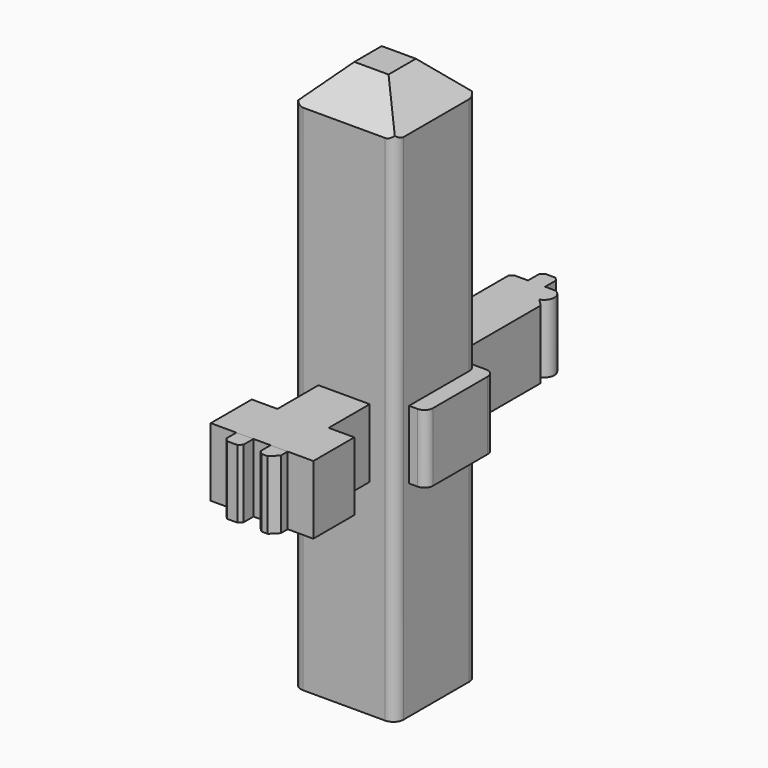
from build123d import *

# Parameters (mm, degrees)
F1_DEPTH      = 25.4
F2_SIZE       = 1.27
F4_DEPTH      = 25.4
F5_SIZE       = 1.27
F6_R          = 3.175
F7_W          = 38.1
F7_H          = 38.1
F8_DEPTH      = 101.6
F9_R          = 3.81
F10_T1_DEPTH  = 95.8007478943
F10_T3_DEPTH  = 95.8007478943
F10_T8_ANGLE  = 90
F10_T13_ANGLE = 90
F10_T18_ANGLE = 90
F10_T23_ANGLE = 90
F10_T28_ANGLE = 90
F10_T33_ANGLE = 90
F10_T38_ANGLE = 90
F10_T43_ANGLE = 90
F12_DEPTH     = 25.4


# Not quite as in the source:
# - a fillet or chamfer that OpenCascade refuses, or shapes differently, is made with other operations: its cross-section is extruded or revolved along the edge and cut away or added


with BuildPart() as f1:
    # F0 (on Top) → F1 (new body)
    with BuildSketch(Plane.XY):
        with BuildLine():
            Line((-3.175, -63.0320869496), (-3.175, -55.4120869496))
            Line((-3.175, -55.4120869496), (3.175, -55.4120869496))
            Line((3.175, -55.4120869496), (3.175, -63.0320869496))
            Line((3.175, -63.0320869496), (6.8309231637, -63.0320869496))
            Line((6.8309231637, -63.0320869496), (9.525, -60.3380101133))
            Line((9.525, -60.3380101133), (9.525, -6.3369898867))
            Line((9.525, -6.3369898867), (6.8309231637, -3.6429130504))
            ThreePointArc((6.8309231637, -3.6429130504), (9.525, 0), (6.8309231637, 3.6429130504))
            Line((6.8309231637, 3.6429130504), (9.525, 6.3369898867))
            Line((9.525, 6.3369898867), (9.525, 60.3380101133))
            Line((9.525, 60.3380101133), (6.8309231637, 63.0320869496))
            ThreePointArc((6.8309231637, 63.0320869496), (9.525, 66.675), (6.8309231637, 70.3179130504))
            Line((6.8309231637, 70.3179130504), (3.175, 70.3179130504))
            Line((3.175, 70.3179130504), (3.175, 76.6679130504))
            Line((3.175, 76.6679130504), (-3.175, 76.6679130504))
            Line((-3.175, 76.6679130504), (-3.175, 70.3179130504))
            Line((-3.175, 70.3179130504), (-9.525, 70.3179130504))
            Line((-9.525, 70.3179130504), (-9.525, -63.0320869496))
            Line((-9.525, -63.0320869496), (-3.175, -63.0320869496))
        make_face()
    extrude(amount=-F1_DEPTH)

    # F2
    f2_edges = [f1.edges().sort_by_distance(p)[0] for p in [
        (-3.175, 76.667913, -12.7),
        (-9.525, 70.317913, -12.7),
        (3.175, 76.667913, -12.7),
        (-9.525, -63.032087, -12.7),
        (-3.175, -63.032087, -12.7),
        (3.175, -63.032087, -12.7),
    ]]
    chamfer(f2_edges, length=F2_SIZE)


with BuildPart() as f4:
    # F3 (on Top) → F4 (new body)
    with BuildSketch(Plane.XY):
        Polygon((0, 19.05), (0, 0), (-12.7, 0), (-12.7, -12.7), (25.4, -12.7), (25.4, 19.05), (12.7, 19.05), (12.7, 25.4), (6.35, 25.4), (6.35, 19.05), align=None)
    extrude(amount=-F4_DEPTH)

    # F5
    f5_edges = [f4.edges().sort_by_distance(p)[0] for p in [
        (12.7, 25.4, -12.7),
        (6.35, 25.4, -12.7),
        (0, 19.05, -12.7),
        (-12.7, 0, -12.7),
    ]]
    chamfer(f5_edges, length=F5_SIZE)

    # F6
    f6_edges = [f4.edges().sort_by_distance(p)[0] for p in [
        (25.4, 19.05, -12.7),
        (25.4, -12.7, -12.7),
    ]]
    fillet(f6_edges, radius=F6_R)


with BuildPart() as f8:
    # F7 (on Top) → F8 (new body, symmetric)
    with BuildSketch(Plane.XY):
        Rectangle(F7_W, F7_H)
    extrude(amount=F8_DEPTH, both=True)

    # F9
    f9_edges = [f8.edges().sort_by_distance(p)[0] for p in [
        (-19.05, -19.05, 0),
        (19.05, -19.05, 0),
        (19.05, 19.05, 0),
        (-19.05, 19.05, 0),
    ]]
    fillet(f9_edges, radius=F9_R)

    # F10: chamfer of 12.7 on 4 edges, made by hand

    # F10_s2 → F10_t1 (cut)
    with BuildSketch(Plane.YZ.offset(-47.9003739472)):
        Polygon((6.35, 101.6), (19.05, 88.9), (19.05, 101.6), align=None)
        Polygon((-19.05, 88.9), (-6.35, 101.6), (-19.05, 101.6), align=None)
    extrude(amount=F10_T1_DEPTH, mode=Mode.SUBTRACT)

    # F10_s4 → F10_t3 (cut)
    with BuildSketch(Plane.XZ.offset(-47.9003739472)):
        Polygon((-6.35, 101.6), (-19.05, 88.9), (-19.05, 101.6), align=None)
        Polygon((6.35, 101.6), (19.05, 88.9), (19.05, 101.6), align=None)
    extrude(amount=F10_T3_DEPTH, mode=Mode.SUBTRACT)


with BuildPart() as f10_tool6:
    # F10_s7 → F10_t8 (revolve)
    with BuildSketch(Plane.YZ.offset(15.24)):
        Polygon((-19.05, 88.9), (-15.24, 92.71), (-15.24, 101.6), (-19.05, 101.6), align=None)
    revolve(axis=Axis((15.24, -15.24, 101.6), (0, 0, 1)), revolution_arc=F10_T8_ANGLE)

    split(bisect_by=Plane(origin=(0, -53.975, 53.975), x_dir=(1, 0, 0), z_dir=(0, -0.7071067812, 0.7071067812)), keep=Keep.TOP)


with BuildPart() as f8_1:
    add(f8.part)

    # F10_t5: cut F10_tool6
    add(f10_tool6.part, mode=Mode.SUBTRACT)


with BuildPart() as f10_tool11:
    # F10_s12 → F10_t13 (revolve)
    with BuildSketch(Plane.YZ.offset(15.24)):
        Polygon((-19.05, 88.9), (-15.24, 92.71), (-15.24, 101.6), (-19.05, 101.6), align=None)
    revolve(axis=Axis((15.24, -15.24, 101.6), (0, 0, 1)), revolution_arc=F10_T13_ANGLE)

    split(bisect_by=Plane(origin=(53.975, 0, 53.975), x_dir=(0, 1, 0), z_dir=(0.7071067812, 0, 0.7071067812)), keep=Keep.TOP)


with BuildPart() as f8_2:
    add(f8_1.part)

    # F10_t10: cut F10_tool11
    add(f10_tool11.part, mode=Mode.SUBTRACT)


with BuildPart() as f10_tool16:
    # F10_s17 → F10_t18 (revolve)
    with BuildSketch(Plane.YZ.offset(15.24)):
        Polygon((15.24, 92.71), (19.05, 88.9), (19.05, 101.6), (15.24, 101.6), align=None)
    revolve(axis=Axis((15.24, 15.24, 101.6), (0, 0, -1)), revolution_arc=F10_T18_ANGLE)

    split(bisect_by=Plane(origin=(0, 53.975, 53.975), x_dir=(1, 0, 0), z_dir=(0, 0.7071067812, 0.7071067812)), keep=Keep.TOP)


with BuildPart() as f8_3:
    add(f8_2.part)

    # F10_t15: cut F10_tool16
    add(f10_tool16.part, mode=Mode.SUBTRACT)


with BuildPart() as f10_tool21:
    # F10_s22 → F10_t23 (revolve)
    with BuildSketch(Plane.YZ.offset(15.24)):
        Polygon((15.24, 92.71), (19.05, 88.9), (19.05, 101.6), (15.24, 101.6), align=None)
    revolve(axis=Axis((15.24, 15.24, 101.6), (0, 0, -1)), revolution_arc=F10_T23_ANGLE)

    split(bisect_by=Plane(origin=(53.975, 0, 53.975), x_dir=(0, 1, 0), z_dir=(0.7071067812, 0, 0.7071067812)), keep=Keep.TOP)


with BuildPart() as f8_4:
    add(f8_3.part)

    # F10_t20: cut F10_tool21
    add(f10_tool21.part, mode=Mode.SUBTRACT)


with BuildPart() as f10_tool26:
    # F10_s27 → F10_t28 (revolve)
    with BuildSketch(Plane.YZ.offset(-15.24)):
        Polygon((-19.05, 88.9), (-15.24, 92.71), (-15.24, 101.6), (-19.05, 101.6), align=None)
    revolve(axis=Axis((-15.24, -15.24, 101.6), (0, 0, -1)), revolution_arc=F10_T28_ANGLE)

    split(bisect_by=Plane(origin=(0, -53.975, 53.975), x_dir=(1, 0, 0), z_dir=(0, -0.7071067812, 0.7071067812)), keep=Keep.TOP)


with BuildPart() as f8_5:
    add(f8_4.part)

    # F10_t25: cut F10_tool26
    add(f10_tool26.part, mode=Mode.SUBTRACT)


with BuildPart() as f10_tool31:
    # F10_s32 → F10_t33 (revolve)
    with BuildSketch(Plane.YZ.offset(-15.24)):
        Polygon((-19.05, 88.9), (-15.24, 92.71), (-15.24, 101.6), (-19.05, 101.6), align=None)
    revolve(axis=Axis((-15.24, -15.24, 101.6), (0, 0, -1)), revolution_arc=F10_T33_ANGLE)

    split(bisect_by=Plane(origin=(-53.975, 0, 53.975), x_dir=(0, 1, 0), z_dir=(-0.7071067812, 0, 0.7071067812)), keep=Keep.TOP)


with BuildPart() as f8_6:
    add(f8_5.part)

    # F10_t30: cut F10_tool31
    add(f10_tool31.part, mode=Mode.SUBTRACT)


with BuildPart() as f10_tool36:
    # F10_s37 → F10_t38 (revolve)
    with BuildSketch(Plane.XZ.offset(-15.24)):
        Polygon((-15.24, 92.71), (-19.05, 88.9), (-19.05, 101.6), (-15.24, 101.6), align=None)
    revolve(axis=Axis((-15.24, 15.24, 101.6), (0, 0, -1)), revolution_arc=F10_T38_ANGLE)

    split(bisect_by=Plane(origin=(-53.975, 0, 53.975), x_dir=(0, 1, 0), z_dir=(-0.7071067812, 0, 0.7071067812)), keep=Keep.TOP)


with BuildPart() as f8_7:
    add(f8_6.part)

    # F10_t35: cut F10_tool36
    add(f10_tool36.part, mode=Mode.SUBTRACT)


with BuildPart() as f10_tool41:
    # F10_s42 → F10_t43 (revolve)
    with BuildSketch(Plane.XZ.offset(-15.24)):
        Polygon((-15.24, 92.71), (-19.05, 88.9), (-19.05, 101.6), (-15.24, 101.6), align=None)
    revolve(axis=Axis((-15.24, 15.24, 101.6), (0, 0, -1)), revolution_arc=F10_T43_ANGLE)

    split(bisect_by=Plane(origin=(0, 53.975, 53.975), x_dir=(1, 0, 0), z_dir=(0, 0.7071067812, 0.7071067812)), keep=Keep.TOP)


with BuildPart() as f8_8:
    add(f8_7.part)

    # F10_t40: cut F10_tool41
    add(f10_tool41.part, mode=Mode.SUBTRACT)


with BuildPart() as f12:
    # F11 (on Top) → F12 (new body)
    with BuildSketch(Plane.XY):
        Polygon((19.05, -57.15), (19.05, -38.1), (9.525, -38.1), (9.525, 0), (-9.525, 0), (-9.525, -38.1), (-19.05, -38.1), (-19.05, -57.15), align=None)
    extrude(amount=-F12_DEPTH)


solid = Compound([f1.part, f4.part, f8_8.part, f12.part])
